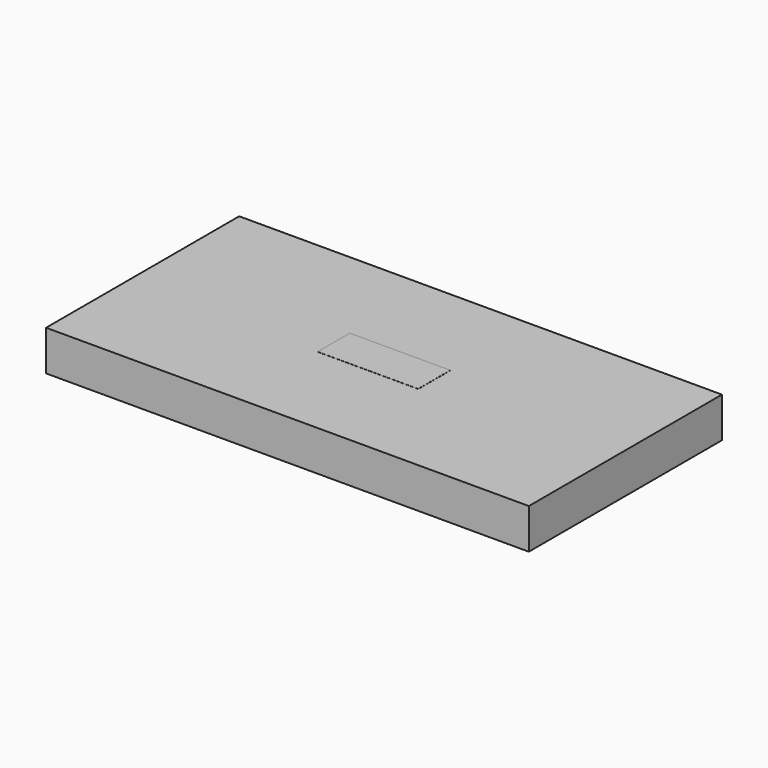
from build123d import *

# Parameters (mm, degrees)
F0_W     = 1219.2
F0_H     = 609.6
F1_DEPTH = 12.7
F2_W     = 38.1
F2_H     = 533.4
F3_DEPTH = 88.9
F4_W     = 254
F4_H     = 101.6
F5_DEPTH = 0.254


# Not quite as in the source:
# - a length typed as a fraction of an inch, garbled in the dataset ("3 / 203.2 mm" for 3/8 in), is restored


with BuildPart() as f1:
    # F0 (on Top) → F1 (new body)
    with BuildSketch(Plane.XY):
        with Locations((-609.6, -177.4520107999)):
            Rectangle(F0_W, F0_H)
    extrude(amount=F1_DEPTH)

    # F2 (on face) → F3 (join)
    with BuildSketch(Plane(origin=(0, 0, 0), x_dir=(1, 0, 0), z_dir=(0, 0, -1))):
        Polygon((-1181.1, -89.2479892001), (-1219.2, -89.2479892001), (-1219.2, -127.3479892001), (0, -127.3479892001), (0, -89.2479892001), (-38.1, -89.2479892001), (-1167.365193367, -89.2479892001), align=None)
        Polygon((0, 482.2520107999), (-1219.2, 482.2520107999), (-1219.2, 444.1520107999), (-1181.1, 444.1520107999), (-1167.365193367, 444.1520107999), (-38.1, 444.1520107999), (0, 444.1520107999), align=None)
        with Locations((-1200.15, 177.4520107999)):
            Rectangle(F2_W, F2_H)
        with Locations((-19.05, 177.4520107999)):
            Rectangle(F2_W, F2_H)
    extrude(amount=F3_DEPTH)

    # F4 (on face) → F5 (join)
    with BuildSketch(Plane.XY.offset(12.7)):
        with Locations((-609.6, -177.4520107999)):
            Rectangle(F4_W, F4_H)
    extrude(amount=F5_DEPTH)


solid = f1.part
